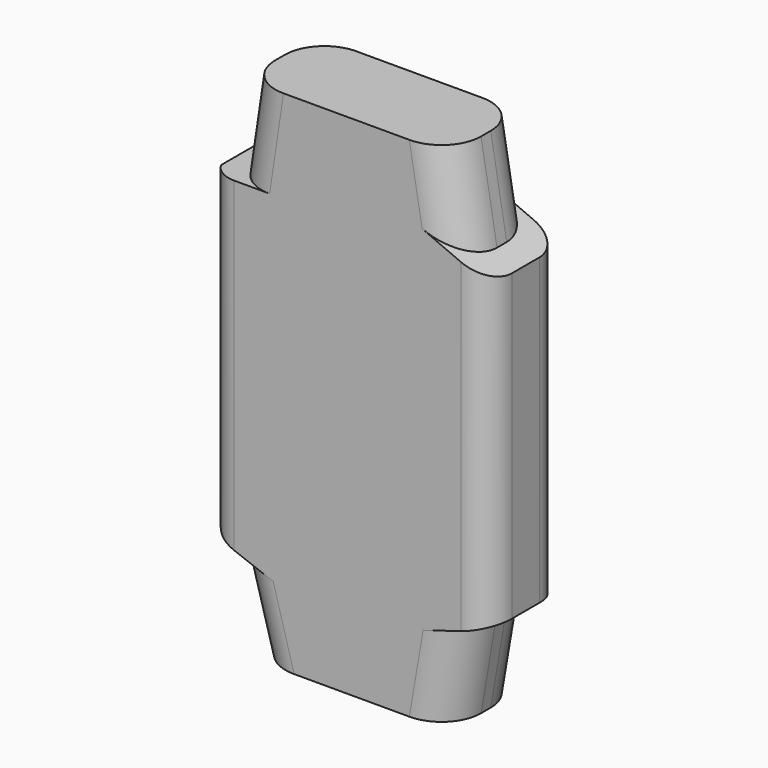
from build123d import *

# Parameters (mm, degrees)
F1_DEPTH    = 2.05
F2_R        = 1.778
F3_T1_DEPTH = 21.8600313558
F3_T3_DEPTH = 20.039287103


# Not quite as in the source:
# - a fillet or chamfer that OpenCascade refuses, or shapes differently, is made with other operations: its cross-section is extruded or revolved along the edge and cut away or added


with BuildPart() as f1:
    # F0 (on Front) → F1 (new body, symmetric)
    with BuildSketch(Plane.XZ):
        with BuildLine():
            Line((10.9602659295, 4.8513999983), (9.6458090239, 4.8513999983))
            add(Edge.make_bspline(
                [(9.6458090239, 4.8513999983), (7.4316049079, 4.8513999983), (5.2174007918, 4.8513999983), (3.0031966758, 4.8513999983)],
                knots=[0, 0, 0, 0, 1, 1, 1, 1], degree=3))
            Line((3.0031966758, 4.8513999983), (1.6934335208, 4.8513999983))
            Line((1.6934335208, 4.8513999983), (1.0692595786, 0.6714852005))
            Line((1.0692595786, 0.6714852005), (0.1693212299, 0.6714852005))
            Line((0.1693212299, 0.6714852005), (-6.1e-09, 0.2293704145))
            Line((-6.1e-09, 0.2293704145), (2.07e-08, -13.0581609413))
            add(Edge.make_bspline(
                [(2.07e-08, -13.0581609413), (0.2048945317, -13.5783853515), (0.7213722482, -13.7736584116)],
                knots=[5.4605557212, 5.4605557212, 5.4605557212, 6.2831853072, 6.2831853072, 6.2831853072], degree=2, weights=[1, 0.9165959415, 1]))
            Line((0.7213722482, -13.7736584116), (0.9610938358, -13.8642938587))
            Line((0.9610938358, -13.8642938587), (2.1238978538, -18.0086))
            Line((2.1238978538, -18.0086), (3.4693217803, -18.0086))
            add(Edge.make_bspline(
                [(9.646094231, -18.0086), (7.5871700808, -18.0086), (5.5282459306, -18.0086), (3.4693217803, -18.0086)],
                knots=[0, 0, 0, 0, 1, 1, 1, 1], degree=3))
            Line((9.646094231, -18.0086), (10.9602659326, -18.0086))
            Line((10.9602659326, -18.0086), (11.6790564953, -13.801625983))
            Line((11.6790564953, -13.801625983), (12.7507999945, -13.4755201564))
            Line((12.7507999945, -13.4755201564), (12.7507999945, 0.2137669466))
            Line((12.7507999945, 0.2137669466), (11.679056502, 0.6762536924))
            Line((11.679056502, 0.6762536924), (10.9602659295, 4.8513999983))
        make_face()
    extrude(amount=F1_DEPTH, both=True)

    # F2
    f2_edges = [f1.edges().sort_by_distance(p)[0] for p in [
        (1.381347, -2.05, 2.761443),
        (1.381347, 2.05, 2.761443),
        (11.319661, -2.05, 2.763827),
        (11.319661, 2.05, 2.763827),
        (11.319661, -2.05, -15.905113),
        (1.542496, -2.05, -15.936447),
        (11.319661, 2.05, -15.905113),
        (1.542496, 2.05, -15.936447),
    ]]
    fillet(f2_edges, radius=F2_R)

    # F3: fillet of radius 1.27 on 4 edges, made by hand

    # F3_s2 → F3_t1 (cut)
    with BuildSketch(Plane.XY.offset(-16.2331609413)):
        with BuildLine():
            ThreePointArc((1.269999983, -2.05), (0.3719743709, -1.6780256121), (-1.7e-08, -0.78))
            Line((-1.7e-08, -0.78), (-1.7e-08, -2.05))
            Line((-1.7e-08, -2.05), (1.269999983, -2.05))
        make_face()
        with BuildLine():
            ThreePointArc((1.269999983, 2.05), (0.3719743709, 1.6780256121), (-1.7e-08, 0.78))
            Line((-1.7e-08, 0.78), (-1.7e-08, 2.05))
            Line((-1.7e-08, 2.05), (1.269999983, 2.05))
        make_face()
    extrude(amount=F3_T1_DEPTH, mode=Mode.SUBTRACT)

    # F3_s4 → F3_t3 (cut)
    with BuildSketch(Plane.XY.offset(-16.6505201564)):
        with BuildLine():
            ThreePointArc((11.4807999945, 2.05), (12.3788256067, 1.6780256121), (12.7507999945, 0.78))
            Line((12.7507999945, 0.78), (12.7507999945, 2.05))
            Line((12.7507999945, 2.05), (11.4807999945, 2.05))
        make_face()
        with BuildLine():
            ThreePointArc((11.4807999945, -2.05), (12.3788256067, -1.6780256121), (12.7507999945, -0.78))
            Line((12.7507999945, -0.78), (12.7507999945, -2.05))
            Line((12.7507999945, -2.05), (11.4807999945, -2.05))
        make_face()
    extrude(amount=F3_T3_DEPTH, mode=Mode.SUBTRACT)


solid = f1.part
